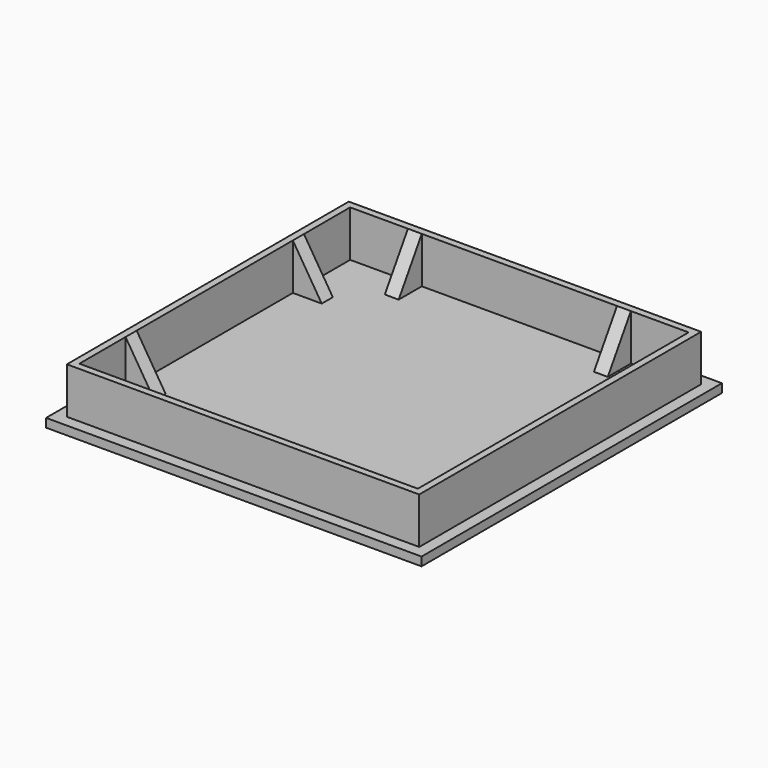
from build123d import *

# Parameters (mm, degrees)
F0_W     = 65
F0_H     = 65
F1_DEPTH = 1.5
F2_W     = 61
F2_H     = 61
F3_DEPTH = 8
F4_SIZE2 = 7.99999
F4_SIZE  = 4.99999


# Not quite as in the source:
# - a fillet or chamfer is up to 0.001 mm smaller than in the source, because OpenCascade refuses the exact size


with BuildPart() as f1:
    # F0 (on Top) → F1 (new body)
    with BuildSketch(Plane.XY):
        Rectangle(F0_W, F0_H)
    extrude(amount=F1_DEPTH)

    # F2 (on face) → F3 (join)
    with BuildSketch(Plane.XY.offset(1.5)):
        Rectangle(F2_W, F2_H)
        Polygon((-29.3, 19.3), (-29.3, 29.3), (-19.3, 29.3), (-19.3, 24.3), (-16.9, 24.3), (-16.9, 29.3), (16.9, 29.3), (16.9, 24.3), (19.3, 24.3), (19.3, 29.3), (29.3, 29.3), (29.3, 19.3), (24.3, 19.3), (24.3, 16.9), (29.3, 16.9), (29.3, -16.9), (24.3, -16.9), (24.3, -19.3), (29.3, -19.3), (29.3, -29.3), (19.3, -29.3), (19.3, -24.3), (16.9, -24.3), (16.9, -29.3), (-16.9, -29.3), (-16.9, -24.3), (-19.3, -24.3), (-19.3, -29.3), (-29.3, -29.3), (-29.3, -19.3), (-24.3, -19.3), (-24.3, -16.9), (-29.3, -16.9), (-29.3, 16.9), (-24.3, 16.9), (-24.3, 19.3), align=None, mode=Mode.SUBTRACT)
    extrude(amount=F3_DEPTH)

    # F4 (size 5 and 8 in the source; OpenCascade refuses exactly that, so slightly less here)
    f4_edges = [f1.edges().sort_by_distance(p)[0] for p in [
        (-24.3, 18.1, 9.5),
        (-18.1, 24.3, 9.5),
        (18.1, 24.3, 9.5),
        (24.3, 18.1, 9.5),
        (-18.1, -24.3, 9.5),
        (-24.3, -18.1, 9.5),
        (18.1, -24.3, 9.5),
        (24.3, -18.1, 9.5),
    ]]
    f4_side = f1.faces().sort_by_distance((0, 29.63733, 9.5))[0]
    chamfer(f4_edges, length=F4_SIZE, length2=F4_SIZE2, reference=f4_side)


solid = f1.part
